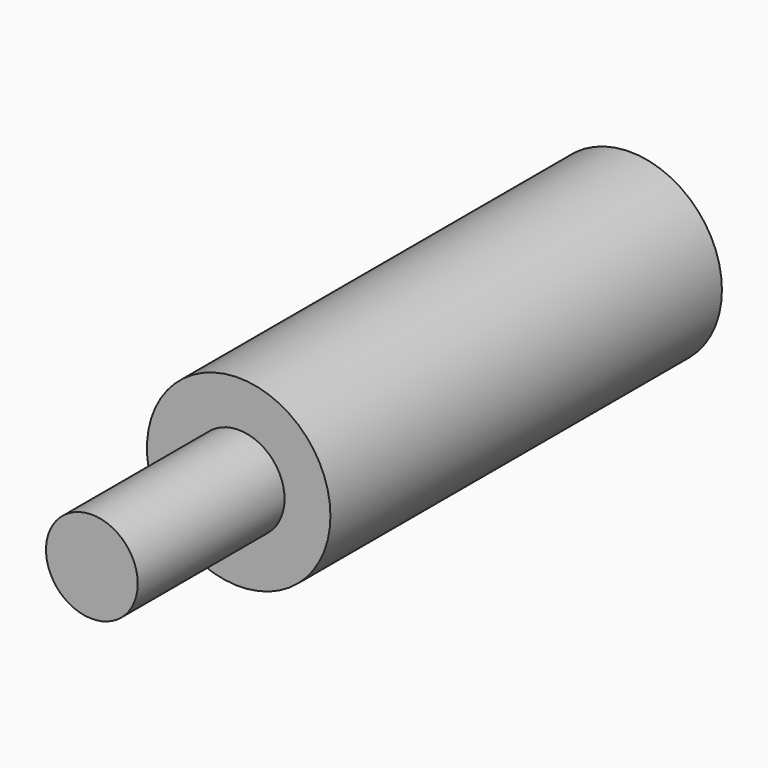
from build123d import *

# Parameters (mm, degrees)
F0_R     = 4.7625
F1_DEPTH = 25.4
F2_R     = 2.38125
F3_DEPTH = 9.525


# Not quite as in the source:
# - a length typed as a fraction of an inch, garbled in the dataset ("3 / 203.2 mm" for 3/8 in), is restored


with BuildPart() as f1:
    # F0 (on Front) → F1 (new body)
    with BuildSketch(Plane.XZ):
        Circle(F0_R)
    extrude(amount=F1_DEPTH)

    # F2 (on face) → F3 (join)
    with BuildSketch(Plane.XZ.offset(25.4)):
        Circle(F2_R)
    extrude(amount=F3_DEPTH)


solid = f1.part
